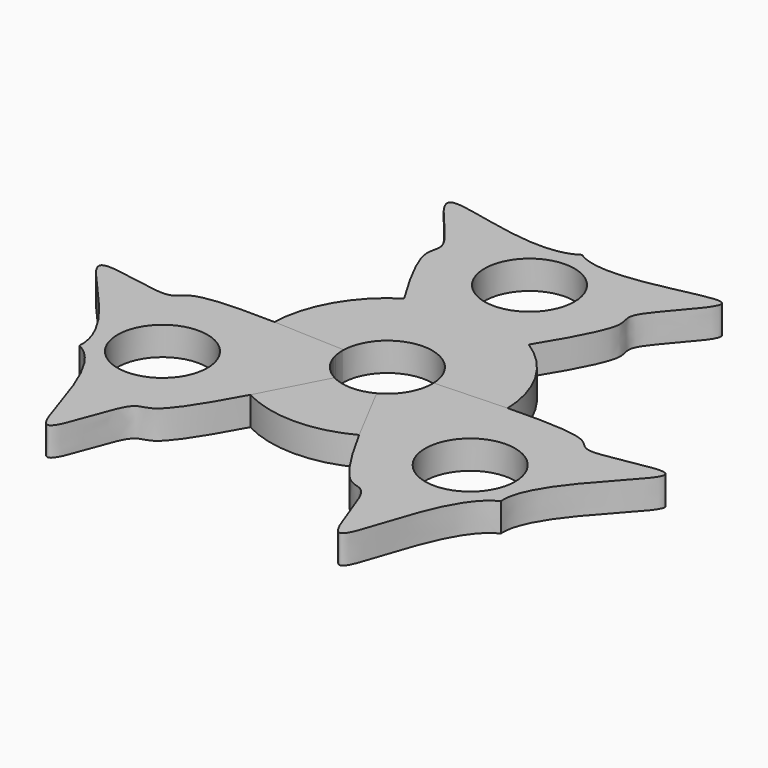
from build123d import *

# Parameters (mm, degrees)
F2_DEPTH = 7
F0_R     = 11.03
F3_DEPTH = 45.6
F4_COUNT = 3
F5_R     = 28.6535577474
F6_DEPTH = 7
F7_DEPTH = 25


with BuildPart() as f2:
    # F1 (on Top) → F2 (new body)
    with BuildSketch(Plane.XY):
        with BuildLine():
            add(Edge.make_bspline(
                [(0, 0), (-9.8764091539, 16.1541642436), (-27.4707564343, 41.0125164581), (-20.3936808927, 46.0300729048), (-47.763111083, 70.4614863935), (-8.9680751782, 53.4871265852), (0, 59.6891157329)],
                knots=[0, 0, 0, 0, 0.300504225, 0.3998907963, 0.5803320288, 0.8320582597, 0.8320582597, 0.8320582597, 0.8320582597], degree=3))
            Line((0, 0), (0, 59.6891157329))
        make_face()
        with BuildLine():
            Line((0, 59.6891157329), (0, 0))
            add(Edge.make_bspline(
                [(0, 0), (9.8764091539, 16.1541642436), (27.4707564343, 41.0125164581), (20.3936808927, 46.0300729048), (47.763111083, 70.4614863935), (8.9680751782, 53.4871265852), (0, 59.6891157329)],
                knots=[0, 0, 0, 0, 0.300504225, 0.3998907963, 0.5803320288, 0.8320582597, 0.8320582597, 0.8320582597, 0.8320582597], degree=3))
        make_face()
    extrude(amount=F2_DEPTH)

    # F0 (on Top) → F3 (cut)
    with BuildSketch(Plane.XY):
        with Locations((0, 43.5798426213)):
            Circle(F0_R)
    extrude(amount=F3_DEPTH, mode=Mode.SUBTRACT)


with BuildPart() as f4_1:
    # F4: instance of F2
    add(f2.part.rotate(Axis((0, 0, 3.5), (0, 0, -1)), 1 * 360 / F4_COUNT))


with BuildPart() as f4_2:
    # F4: instance of F2
    add(f2.part.rotate(Axis((0, 0, 3.5), (0, 0, -1)), 2 * 360 / F4_COUNT))


with BuildPart() as f2_1:
    add(f2.part)

    # F5 (on Top) → F6 (join)
    with BuildSketch(Plane.XY):
        Circle(F5_R)
    extrude(amount=F6_DEPTH)


with BuildPart() as f7_tool:
    # F0 (on Top) → F7 (new body)
    with BuildSketch(Plane.XY):
        Circle(F0_R)
    extrude(amount=F7_DEPTH)


with BuildPart() as f2_2:
    add(f2_1.part)

    # F7: cut by f7_tool
    add(f7_tool.part, mode=Mode.SUBTRACT)


with BuildPart() as f4_1_1:
    add(f4_1.part)

    # F7: cut by f7_tool
    add(f7_tool.part, mode=Mode.SUBTRACT)


with BuildPart() as f4_2_1:
    add(f4_2.part)

    # F7: cut by f7_tool
    add(f7_tool.part, mode=Mode.SUBTRACT)


solid = Compound([f2_2.part, f4_1_1.part, f4_2_1.part])
